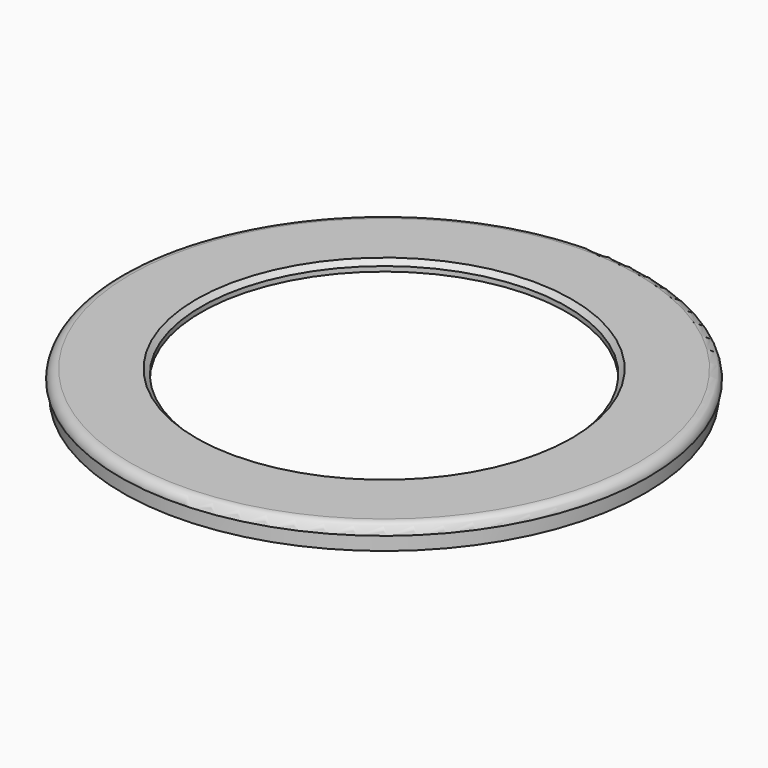
from build123d import *

# Parameters (mm, degrees)
F0_R     = 53.4294983316
F0_R_2   = 51.6
F1_DEPTH = 3
F3_R     = 53.9566734819
F4_DEPTH = 2
F5_R     = 1.99999
F6_R     = 37.4035262833
F7_DEPTH = 3
F8_SIZE2 = 1
F8_SIZE  = 1


# Not quite as in the source:
# - a fillet or chamfer is up to 0.001 mm smaller than in the source, because OpenCascade refuses the exact size


with BuildPart() as f1:
    # F0 (on Top) → F1 (new body)
    with BuildSketch(Plane.XY):
        Circle(F0_R)
        Circle(F0_R_2, mode=Mode.SUBTRACT)
    extrude(amount=-F1_DEPTH)

    # F3 (on offset) → F4 (join)
    with BuildSketch(Plane.XY):
        Circle(F3_R)
    extrude(amount=F4_DEPTH)

    # F5 (radius 2 in the source; OpenCascade refuses exactly that, so slightly less here)
    f5_edges = [f1.edges().sort_by_distance(p)[0] for p in [
        (-53.956673, 0, 2),
    ]]
    fillet(f5_edges, radius=F5_R)

    # F6 (on offset) → F7 (cut)
    with BuildSketch(Plane.XY):
        Circle(F6_R)
    extrude(amount=F7_DEPTH, mode=Mode.SUBTRACT)

    # F8
    f8_edges = [f1.edges().sort_by_distance(p)[0] for p in [
        (-37.403526, 0, 2),
    ]]
    chamfer(f8_edges, length=F8_SIZE, length2=F8_SIZE2)


solid = f1.part
